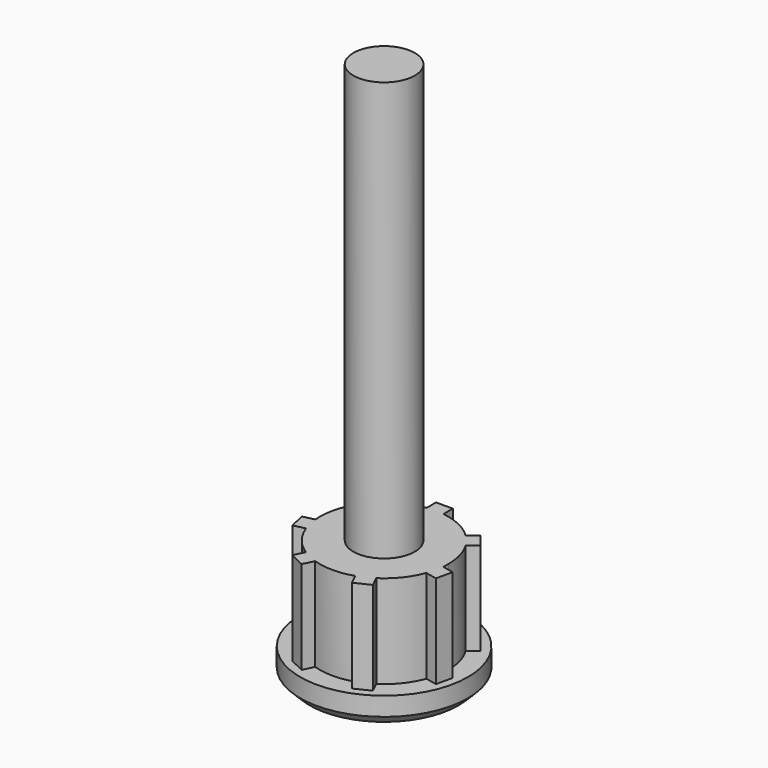
from build123d import *

# Parameters (mm, degrees)
F0_R     = 11.43
F1_DEPTH = 3.81
F3_DEPTH = 12.7
F4_R     = 4.191
F5_DEPTH = 57.15
F6_DEPTH = 57.15
F7_SIZE  = 1.27
F8_DEPTH = 12.7


with BuildPart() as f1:
    # F0 (on Top) → F1 (new body)
    with BuildSketch(Plane.XY):
        Circle(F0_R)
    extrude(amount=F1_DEPTH)

    # F2 (on face) → F3 (join)
    with BuildSketch(Plane.XY.offset(3.81)):
        with BuildLine():
            ThreePointArc((8.7246484395, -0.8189496979), (8.7534068589, -0.4099236057), (8.763, 0))
            ThreePointArc((8.763, 0), (8.4427240898, 2.3474622346), (7.5053076703, 4.5233312696))
            ThreePointArc((7.5053076703, 4.5233312696), (6.8511892809, 5.4636411337), (6.0800099832, 6.3105980385))
            ThreePointArc((6.0800099832, 6.3105980385), (3.8021232059, 7.8951901894), (1.143, 8.6881367393))
            ThreePointArc((1.143, 8.6881367393), (0, 8.763), (-1.143, 8.6881367393))
            ThreePointArc((-1.143, 8.6881367393), (-3.8021232059, 7.8951901894), (-6.0800099832, 6.3105980385))
            ThreePointArc((-6.0800099832, 6.3105980385), (-6.8511892809, 5.4636411337), (-7.5053076703, 4.5233312696))
            ThreePointArc((-7.5053076703, 4.5233312696), (-8.5432932944, 1.9499509443), (-8.7246484395, -0.8189496979))
            ThreePointArc((-8.7246484395, -0.8189496979), (-8.5432932944, -1.9499509443), (-8.2159655844, -3.0476349052))
            ThreePointArc((-8.2159655844, -3.0476349052), (-6.8511892809, -5.4636411337), (-4.7994486704, -7.3318116083))
            ThreePointArc((-4.7994486704, -7.3318116083), (-3.8021232059, -7.8951901894), (-2.7398338384, -8.323669836))
            ThreePointArc((-2.7398338384, -8.323669836), (0, -8.763), (2.7398338384, -8.323669836))
            ThreePointArc((2.7398338384, -8.323669836), (3.8021232059, -7.8951901894), (4.7994486704, -7.3318116083))
            ThreePointArc((4.7994486704, -7.3318116083), (6.8511892809, -5.4636411337), (8.2159655844, -3.0476349052))
            ThreePointArc((8.2159655844, -3.0476349052), (8.5432932944, -1.9499509443), (8.7246484395, -0.8189496979))
        make_face()
    extrude(amount=F3_DEPTH)

    # F4 (on face) → F5 (join)
    with BuildSketch(Plane.XY.offset(16.51)):
        Circle(F4_R)
    extrude(amount=F5_DEPTH)

    # F4 (on face) → F6 (join)
    with BuildSketch(Plane.XY.offset(16.51)):
        Circle(F4_R)
    extrude(amount=F6_DEPTH)

    # F7
    f7_edges = [f1.edges().sort_by_distance(p)[0] for p in [
        (-11.43, 0, 0),
    ]]
    chamfer(f7_edges, length=F7_SIZE)

    # F2 (on face) → F8 (join)
    with BuildSketch(Plane.XY.offset(3.81)):
        with BuildLine():
            ThreePointArc((8.7246484395, -0.8189496979), (8.7534068589, -0.4099236057), (8.763, 0))
            ThreePointArc((8.763, 0), (8.4427240898, 2.3474622346), (7.5053076703, 4.5233312696))
            ThreePointArc((7.5053076703, 4.5233312696), (6.8511892809, 5.4636411337), (6.0800099832, 6.3105980385))
            ThreePointArc((6.0800099832, 6.3105980385), (3.8021232059, 7.8951901894), (1.143, 8.6881367393))
            ThreePointArc((1.143, 8.6881367393), (0, 8.763), (-1.143, 8.6881367393))
            ThreePointArc((-1.143, 8.6881367393), (-3.8021232059, 7.8951901894), (-6.0800099832, 6.3105980385))
            ThreePointArc((-6.0800099832, 6.3105980385), (-6.8511892809, 5.4636411337), (-7.5053076703, 4.5233312696))
            ThreePointArc((-7.5053076703, 4.5233312696), (-8.5432932944, 1.9499509443), (-8.7246484395, -0.8189496979))
            ThreePointArc((-8.7246484395, -0.8189496979), (-8.5432932944, -1.9499509443), (-8.2159655844, -3.0476349052))
            ThreePointArc((-8.2159655844, -3.0476349052), (-6.8511892809, -5.4636411337), (-4.7994486704, -7.3318116083))
            ThreePointArc((-4.7994486704, -7.3318116083), (-3.8021232059, -7.8951901894), (-2.7398338384, -8.323669836))
            ThreePointArc((-2.7398338384, -8.323669836), (0, -8.763), (2.7398338384, -8.323669836))
            ThreePointArc((2.7398338384, -8.323669836), (3.8021232059, -7.8951901894), (4.7994486704, -7.3318116083))
            ThreePointArc((4.7994486704, -7.3318116083), (6.8511892809, -5.4636411337), (8.2159655844, -3.0476349052))
            ThreePointArc((8.2159655844, -3.0476349052), (8.5432932944, -1.9499509443), (8.7246484395, -0.8189496979))
        make_face()
        with BuildLine():
            ThreePointArc((6.0800099832, 6.3105980385), (6.8511892809, 5.4636411337), (7.5053076703, 4.5233312696))
            Line((7.5053076703, 4.5233312696), (8.7553493037, 5.5202062073))
            Line((8.7553493037, 5.5202062073), (7.3300516166, 7.3074729762))
            Line((7.3300516166, 7.3074729762), (6.0800099832, 6.3105980385))
        make_face()
        with BuildLine():
            Line((10.2834248601, -1.174730244), (8.7246484395, -0.8189496979))
            ThreePointArc((8.7246484395, -0.8189496979), (8.5432932944, -1.9499509443), (8.2159655844, -3.0476349052))
            Line((8.2159655844, -3.0476349052), (9.7747420051, -3.4034154512))
            Line((9.7747420051, -3.4034154512), (10.2834248601, -1.174730244))
        make_face()
        with BuildLine():
            ThreePointArc((-1.143, 8.6881367393), (0, 8.763), (1.143, 8.6881367393))
            Line((1.143, 8.6881367393), (1.143, 10.287))
            Line((1.143, 10.287), (-1.143, 10.287))
            Line((-1.143, 10.287), (-1.143, 8.6881367393))
        make_face()
        with BuildLine():
            Line((5.4931694403, -8.7723376303), (4.7994486704, -7.3318116083))
            ThreePointArc((4.7994486704, -7.3318116083), (3.8021232059, -7.8951901894), (2.7398338384, -8.323669836))
            Line((2.7398338384, -8.323669836), (3.4335546083, -9.7641958579))
            Line((3.4335546083, -9.7641958579), (5.4931694403, -8.7723376303))
        make_face()
        with BuildLine():
            ThreePointArc((-7.5053076703, 4.5233312696), (-6.8511892809, 5.4636411337), (-6.0800099832, 6.3105980385))
            Line((-6.0800099832, 6.3105980385), (-7.3300516166, 7.3074729762))
            Line((-7.3300516166, 7.3074729762), (-8.7553493037, 5.5202062073))
            Line((-8.7553493037, 5.5202062073), (-7.5053076703, 4.5233312696))
        make_face()
        with BuildLine():
            Line((-3.4335546083, -9.7641958579), (-2.7398338384, -8.323669836))
            ThreePointArc((-2.7398338384, -8.323669836), (-3.8021232059, -7.8951901894), (-4.7994486704, -7.3318116083))
            Line((-4.7994486704, -7.3318116083), (-5.4931694403, -8.7723376303))
            Line((-5.4931694403, -8.7723376303), (-3.4335546083, -9.7641958579))
        make_face()
        with BuildLine():
            ThreePointArc((-8.2159655844, -3.0476349052), (-8.5432932944, -1.9499509443), (-8.7246484395, -0.8189496979))
            Line((-8.7246484395, -0.8189496979), (-10.2834248601, -1.174730244))
            Line((-10.2834248601, -1.174730244), (-9.7747420051, -3.4034154512))
            Line((-9.7747420051, -3.4034154512), (-8.2159655844, -3.0476349052))
        make_face()
    extrude(amount=F8_DEPTH)


solid = f1.part
